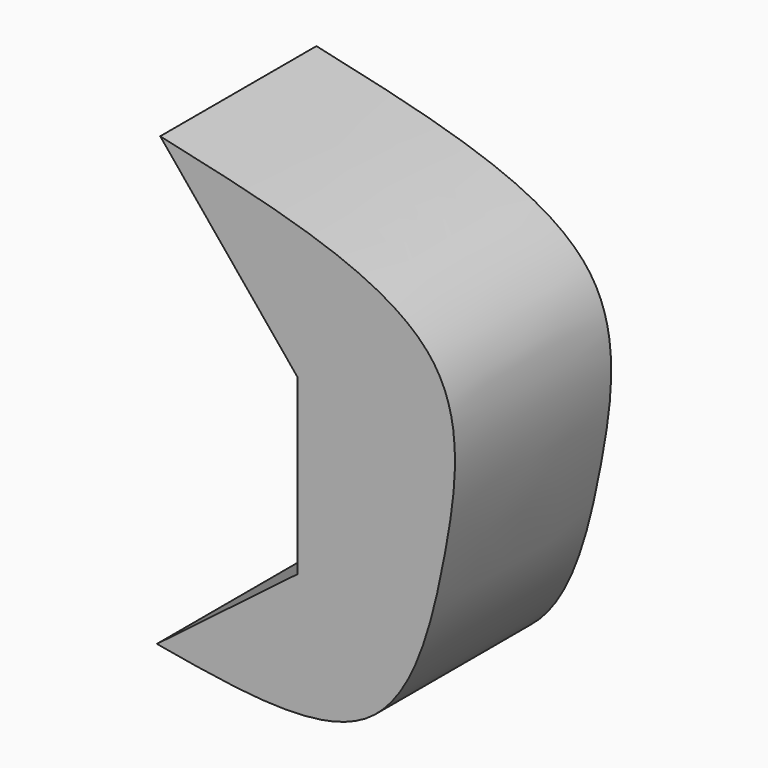
from build123d import *

# Parameters (mm, degrees)
F3_DEPTH = 13.97


# Not quite as in the source:
# - the program builds the solid bodies; features that only make, move or delete a surface that nothing else refers to are left out


with BuildPart() as f3:
    # F2 (on Front) → F3 (new body)
    with BuildSketch(Plane.XZ):
        with BuildLine():
            add(Edge.make_bspline(
                [(30.1382970065, 53.6987893283), (38.2641649903, 51.9034280628), (52.6177925395, 48.7320810789), (50.7954811422, 33.8717910312), (46.8605959622, 18.6504889659), (35.6789275104, 20.6258726517), (29.8991017044, 21.6469522566)],
                knots=[0, 0, 0, 0, 0.2930899362, 0.5177174662, 0.750707236, 1, 1, 1, 1], degree=3))
            Line((30.1382970065, 53.6987893283), (39.9452000856, 41.7391508818))
            Line((39.9452000856, 41.7391508818), (39.9452000856, 29.3011236936))
            Line((39.9452000856, 29.3011236936), (29.8991017044, 21.6469522566))
        make_face()
    extrude(amount=F3_DEPTH)


solid = f3.part
